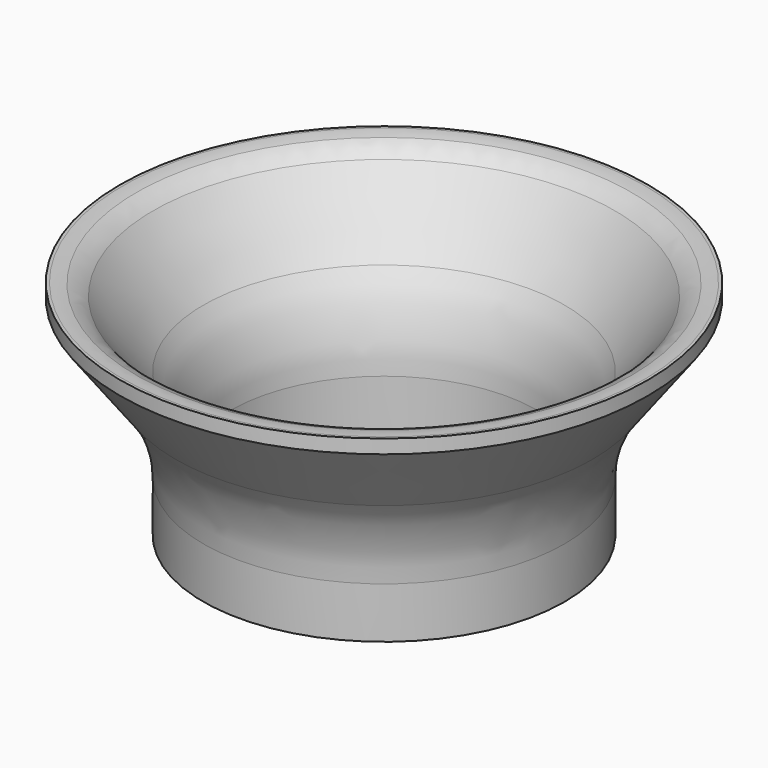
from build123d import *

# Parameters (mm, degrees)
F0_R      = 13
F3_DEPTH  = 7
F2_R      = 19
F4_DEPTH  = 1
F3_FACE_R = 13
F4_FACE_R = 19
F6_T      = -2
F7_R      = 10
F9_R      = 10
F10_R     = 2


# Not quite as in the source:
# - a fillet or chamfer that OpenCascade refuses, or shapes differently, is made with other operations: its cross-section is extruded or revolved along the edge and cut away or added


with BuildPart() as f3:
    # F0 (on Top) → F3 (new body)
    with BuildSketch(Plane.XY):
        Circle(F0_R)
    extrude(amount=F3_DEPTH)



with BuildPart() as f4:
    # F2 (on offset) → F4 (new body)
    with BuildSketch(Plane.XY.offset(15)):
        Circle(F2_R)
    extrude(amount=F4_DEPTH)


with BuildPart() as f3_1:
    add(f3.part)

    add(f4.part)  # F5 merges F4
    # F3_face (on face) → F5 section 0
    with BuildSketch(Plane.XY.offset(7)):
        Circle(F3_FACE_R)
    # F4_face (on face) → F5 section 1
    with BuildSketch(Plane(origin=(0, 0, 15), x_dir=(1, 0, 0), z_dir=(0, 0, -1))):
        Circle(F4_FACE_R)
    loft()

    # F6
    f6_openings = [f3_1.faces().sort_by_distance(p)[0] for p in [
        (0, 0, 16),
        (0, 0, 0),
    ]]
    offset(amount=F6_T, openings=f6_openings, kind=Kind.INTERSECTION)

    # F7
    f7_edges = [f3_1.edges().sort_by_distance(p)[0] for p in [
        (-13, 0, 7),
    ]]
    fillet(f7_edges, radius=F7_R)

    # F8: fillet of radius 5 on 2 edges, made by hand

    # F8_s1 → F8_t2 (revolve, cut)
    with BuildSketch(Plane.XZ):
        with BuildLine():
            ThreePointArc((18.7950549357, 16), (17.8821840065, 15.9159604013), (17, 15.6666666667))
            Line((17, 15.6666666667), (17, 16))
            Line((17, 16), (18.7950549357, 16))
        make_face()
    revolve(axis=Axis((0, 0, 16), (0, 0, -1)), mode=Mode.SUBTRACT)

    # F9
    f9_edges = [f3_1.edges().sort_by_distance(p)[0] for p in [
        (-11, 0, 7.666667),
    ]]
    fillet(f9_edges, radius=F9_R)

    # F10
    f10_edges = [f3_1.edges().sort_by_distance(p)[0] for p in [
        (-17, 0, 15.666667),
    ]]
    fillet(f10_edges, radius=F10_R)


solid = f3_1.part
